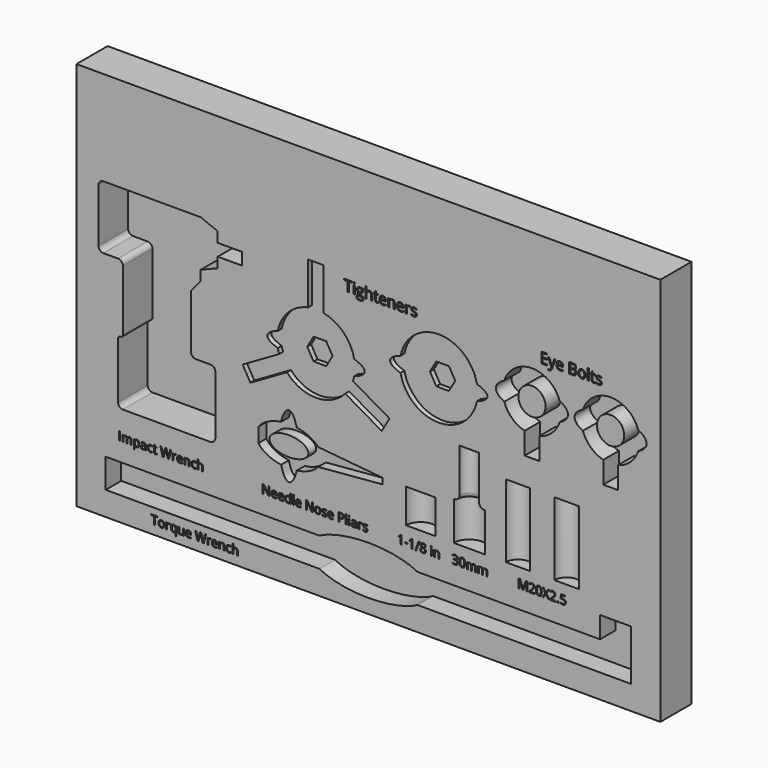
from build123d import *

# Parameters (mm, degrees)
F0_W            = 762
F0_H            = 355.6
F1_DEPTH        = 50.8
F2_R            = 17.78
F3_DEPTH        = 25.4
F0_H_2          = 152.4
F5_DEPTH        = 50.8
F7_DEPTH        = 48.26
F8_DEPTH        = 6.35
F9_DEPTH        = 12.7
F11_DEPTH       = 12.7
F12_DEPTH       = 6.35
F13_DEPTH       = 12.7
F14_TEXT_SIZE   = 15.875
F14_TEXT_SIZE_2 = 19.4027777778
F15_DEPTH       = 3.81
F20_DEPTH       = 12.7
F2_W            = 12.7
F2_H            = 63.5
F22_R           = 6.35


# Not quite as in the source:
# - Text() gives the source's letters only with a copy of the font that has no kerning and outlines rounded to 1/6400 em; it was checked with that copy


with BuildPart() as f1:
    # F0 (on Front) → F1 (new body)
    with BuildSketch(Plane.XZ):
        Rectangle(F0_W, F0_H)
    extrude(amount=F1_DEPTH)

    # F2 (on face) → F3 (cut)
    with BuildSketch(Plane.XZ.offset(50.8)):
        with BuildLine():
            Line((302.26, -80.5533003902), (302.26, -108.4933003902))
            Line((302.26, -108.4933003902), (64.0476572037, -108.4933003902))
            add(Edge.make_bspline(
                [(64.0476572037, -108.4933003902), (0, -74.6266337236), (-64.0476572037, -108.4933003902)],
                knots=[3.7850937624, 3.7850937624, 3.7850937624, 5.6396841984, 5.6396841984, 5.6396841984], degree=2, weights=[1, 0.6, 1]))
            Line((-64.0476572037, -108.4933003902), (-342.9, -108.4933003902))
            Line((-342.9, -108.4933003902), (-342.9, -146.5933003902))
            Line((-342.9, -146.5933003902), (-64.0476572037, -146.5933003902))
            add(Edge.make_bspline(
                [(-64.0476572037, -146.5933003902), (0, -180.4599670569), (64.0476572037, -146.5933003902)],
                knots=[0.6435011088, 0.6435011088, 0.6435011088, 2.4980915448, 2.4980915448, 2.4980915448], degree=2, weights=[1, 0.6, 1]))
            Line((64.0476572037, -146.5933003902), (302.26, -146.5933003902))
            Line((302.26, -146.5933003902), (322.58, -146.5933003902))
            Line((322.58, -146.5933003902), (322.58, -80.5533003902))
            Line((322.58, -80.5533003902), (302.26, -80.5533003902))
        make_face()
        with BuildLine():
            Line((325.5514520794, 70.534063589), (325.5514520794, 99.109063589))
            ThreePointArc((325.5514520794, 99.109063589), (341.9633701455, 108.0906957609), (352.1212254393, 123.8017984246))
            add(Edge.make_bspline(
                [(352.1212254393, 123.8017984246), (377.2004087071, 135.9992299616), (352.1212254393, 148.1966614987)],
                knots=[5.5883159153, 5.5883159153, 5.5883159153, 6.9780546991, 6.9780546991, 6.9780546991], degree=2, weights=[1, 0.7681373347, 1]))
            ThreePointArc((352.1212254393, 148.1966614987), (316.0264520794, 174.0992299616), (279.9316787196, 148.1966614987))
            add(Edge.make_bspline(
                [(279.9316787196, 148.1966614987), (254.8524954518, 135.9992299616), (279.9316787196, 123.8017984246)],
                knots=[2.4467232617, 2.4467232617, 2.4467232617, 3.8364620455, 3.8364620455, 3.8364620455], degree=2, weights=[1, 0.7681373347, 1]))
            ThreePointArc((279.9316787196, 123.8017984246), (290.0895340134, 108.0906957609), (306.5014520794, 99.109063589))
            Line((306.5014520794, 99.109063589), (306.5014520794, 70.534063589))
            Line((306.5014520794, 70.534063589), (316.0264520794, 70.534063589))
            Line((316.0264520794, 70.534063589), (325.5514520794, 70.534063589))
        make_face()
        with BuildLine():
            ThreePointArc((316.0264520794, 118.2192299616), (303.4540935099, 148.5715885311), (333.8064520794, 135.9992299616))
            ThreePointArc((333.8064520794, 135.9992299616), (328.5988106489, 123.4268713921), (316.0264520794, 118.2192299616))
        make_face(mode=Mode.SUBTRACT)
        with BuildLine():
            Line((222.9323361307, 70.534063589), (222.9323361307, 99.109063589))
            ThreePointArc((222.9323361307, 99.109063589), (239.3442541968, 108.0906957609), (249.5021094906, 123.8017984246))
            add(Edge.make_bspline(
                [(249.5021094906, 123.8017984246), (274.5812927584, 135.9992299616), (249.5021094906, 148.1966614987)],
                knots=[2.4467232617, 2.4467232617, 2.4467232617, 3.8364620455, 3.8364620455, 3.8364620455], degree=2, weights=[1, 0.7681373347, 1]))
            ThreePointArc((249.5021094906, 148.1966614987), (213.4073361307, 174.0992299616), (177.3125627709, 148.1966614987))
            add(Edge.make_bspline(
                [(177.3125627709, 148.1966614987), (152.2333795031, 135.9992299616), (177.3125627709, 123.8017984246)],
                knots=[5.5883159153, 5.5883159153, 5.5883159153, 6.9780546991, 6.9780546991, 6.9780546991], degree=2, weights=[1, 0.7681373347, 1]))
            ThreePointArc((177.3125627709, 123.8017984246), (187.4704180647, 108.0906957609), (203.8823361307, 99.109063589))
            Line((203.8823361307, 99.109063589), (203.8823361307, 70.534063589))
            Line((203.8823361307, 70.534063589), (213.4073361307, 70.534063589))
            Line((213.4073361307, 70.534063589), (222.9323361307, 70.534063589))
        make_face()
        with Locations((213.4073361307, 135.9992299616)):
            Circle(F2_R, mode=Mode.SUBTRACT)
        Polygon((342.9, -80.5533003902), (322.58, -80.5533003902), (322.58, -146.5933003902), (342.9, -146.5933003902), (342.9, -108.4933003902), align=None)
    extrude(amount=-F3_DEPTH, mode=Mode.SUBTRACT)

    # F0 (on Front) → F5 (join)
    with BuildSketch(Plane.XZ):
        with Locations((0, 254)):
            Rectangle(F0_W, F0_H_2)
    extrude(amount=F5_DEPTH)

    # F6 (on face) → F7 (cut)
    with BuildSketch(Plane.XZ.offset(50.8)):
        with BuildLine():
            Line((-218.8787088156, 206.9589091301), (-345.8787088156, 206.9589091301))
            ThreePointArc((-345.8787088156, 206.9589091301), (-350.3688368761, 205.0990371906), (-352.2287088156, 200.6089091301))
            Line((-352.2287088156, 200.6089091301), (-352.2287088156, 130.7589091301))
            ThreePointArc((-352.2287088156, 130.7589091301), (-350.3688368761, 126.2687810696), (-345.8787088156, 124.4089091301))
            Line((-345.8787088156, 124.4089091301), (-326.8287088156, 124.4089091301))
            ThreePointArc((-326.8287088156, 124.4089091301), (-322.338580755, 122.5490371906), (-320.4787088156, 118.0589091301))
            Line((-320.4787088156, 118.0589091301), (-320.4787088156, 38.6839091301))
            ThreePointArc((-320.4787088156, 38.6839091301), (-321.4086447853, 36.4388450998), (-323.6537088156, 35.5089091301))
            ThreePointArc((-323.6537088156, 35.5089091301), (-325.8987728458, 34.5789731604), (-326.8287088156, 32.3339091301))
            Line((-326.8287088156, 32.3339091301), (-326.8287088156, -40.6910908699))
            ThreePointArc((-326.8287088156, -40.6910908699), (-324.9688368761, -45.1812189304), (-320.4787088156, -47.0410908699))
            Line((-320.4787088156, -47.0410908699), (-206.1787088156, -47.0410908699))
            ThreePointArc((-206.1787088156, -47.0410908699), (-201.688580755, -45.1812189304), (-199.8287088156, -40.6910908699))
            Line((-199.8287088156, -40.6910908699), (-199.8287088156, 35.5089091301))
            ThreePointArc((-199.8287088156, 35.5089091301), (-201.688580755, 39.9990371906), (-206.1787088156, 41.8589091301))
            Line((-206.1787088156, 41.8589091301), (-225.2287088156, 41.8589091301))
            ThreePointArc((-225.2287088156, 41.8589091301), (-229.7188368761, 43.7187810696), (-231.5787088156, 48.2089091301))
            Line((-231.5787088156, 48.2089091301), (-231.5787088156, 118.0589091301))
            Line((-231.5787088156, 118.0589091301), (-218.8787088156, 133.9339091301))
            Line((-218.8787088156, 133.9339091301), (-218.8787088156, 146.6339091301))
            Line((-218.8787088156, 146.6339091301), (-196.6537088156, 155.5239091301))
            Line((-196.6537088156, 155.5239091301), (-196.6537088156, 168.8589091301))
            Line((-196.6537088156, 168.8589091301), (-164.9037088156, 168.8589091301))
            Line((-164.9037088156, 168.8589091301), (-164.9037088156, 184.7339091301))
            Line((-164.9037088156, 184.7339091301), (-196.6537088156, 184.7339091301))
            Line((-196.6537088156, 184.7339091301), (-196.6537088156, 198.0689091301))
            Line((-196.6537088156, 198.0689091301), (-218.8787088156, 206.9589091301))
        make_face()
    extrude(amount=-F7_DEPTH, mode=Mode.SUBTRACT)

    # F6 (on face) → F8 (cut)
    with BuildSketch(Plane.XZ.offset(50.8)):
        with BuildLine():
            add(Edge.make_bspline(
                [(-118.2285690843, 109.0660422975), (-149.2966618743, 99.2286645982), (-118.2285690843, 89.3912868988)],
                knots=[2.4732611299, 2.4732611299, 2.4732611299, 3.8099241773, 3.8099241773, 3.8099241773], degree=2, weights=[1, 0.7848566748, 1]))
            ThreePointArc((-118.2285690843, 89.3912868988), (-117.4795035517, 86.1566580811), (-116.520739255, 82.9778699814))
            Line((-116.520739255, 82.9778699814), (-164.1237066018, 55.4942839694))
            Line((-164.1237066018, 55.4942839694), (-159.0437066018, 46.695465867))
            Line((-159.0437066018, 46.695465867), (-153.9637066018, 37.8966477645))
            Line((-153.9637066018, 37.8966477645), (-106.3012300457, 65.4145914345))
            ThreePointArc((-106.3012300457, 65.4145914345), (-68.2183829259, 48.4289550604), (-30.2512847531, 65.6717664354))
            Line((-30.2512847531, 65.6717664354), (17.3516825938, 38.1881804235))
            Line((17.3516825938, 38.1881804235), (22.4316825938, 46.9869985259))
            Line((22.4316825938, 46.9869985259), (27.5116825938, 55.7858166284))
            Line((27.5116825938, 55.7858166284), (-20.1507939623, 83.3037602983))
            ThreePointArc((-20.1507939623, 83.3037602983), (-19.2569127775, 86.3227352727), (-18.5517713829, 89.3912868988))
            add(Edge.make_bspline(
                [(-18.5517713829, 89.3912868988), (12.5163214072, 99.2286645982), (-18.5517713829, 109.0660422975)],
                knots=[5.6148537835, 5.6148537835, 5.6148537835, 6.9515168309, 6.9515168309, 6.9515168309], degree=2, weights=[1, 0.7848566748, 1]))
            ThreePointArc((-18.5517713829, 109.0660422975), (-32.4135637837, 135.0940209794), (-58.3984866927, 149.0363573777))
            Line((-58.3984866927, 149.0363573777), (-58.3984866927, 204.0035294015))
            Line((-58.3984866927, 204.0035294015), (-68.5584866927, 204.0035294015))
            Line((-68.5584866927, 204.0035294015), (-78.7184866927, 204.0035294015))
            Line((-78.7184866927, 204.0035294015), (-78.7184866927, 148.9676420617))
            ThreePointArc((-78.7184866927, 148.9676420617), (-104.4878546985, 134.9721559815), (-118.2285690843, 109.0660422975))
        make_face()
        Polygon((-68.3901702336, 113.5161748096), (-60.1242022144, 113.5062921219), (-51.8923980827, 99.2089400686), (-60.1583661018, 84.9313125448), (-76.6561382527, 84.9510370744), (-84.8879423845, 99.2483891277), (-76.6219743653, 113.5260166515), align=None, mode=Mode.SUBTRACT)
    extrude(amount=-F8_DEPTH, mode=Mode.SUBTRACT)

    # F6 (on face) → F9 (cut)
    with BuildSketch(Plane.XZ.offset(50.8)):
        Polygon((-51.8923980827, 99.2089400686), (-60.1242022144, 113.5062921219), (-68.3901702336, 113.5161748096), (-76.6219743653, 113.5260166515), (-84.8879423845, 99.2483891277), (-76.6561382527, 84.9510370744), (-60.1583661018, 84.9313125448), align=None)
    extrude(amount=-F9_DEPTH, mode=Mode.SUBTRACT)

    # F10 (on face) → F11 (cut)
    with BuildSketch(Plane.XZ.offset(50.8)):
        with BuildLine():
            Line((-65.5816475336, -30.0850472887), (18.5110562313, -22.833929086))
            Line((18.5110562313, -22.833929086), (18.5110562313, -19.023929086))
            Line((18.5110562313, -19.023929086), (18.5110562313, -15.213929086))
            Line((18.5110562313, -15.213929086), (-65.5816475336, -7.2250472887))
            add(Edge.make_bspline(
                [(-65.5816475336, -7.2250472887), (-74.4495671038, 3.2276411288), (-93.5893307929, 6.0144929834)],
                knots=[0.466765339, 0.466765339, 0.466765339, 1.3303918197, 1.3303918197, 1.3303918197], degree=2, weights=[1, 0.9082083689, 1]))
            add(Edge.make_bspline(
                [(-93.5893307929, 6.0144929834), (-103.7712937651, 50.4028113586), (-113.9532567372, 6.0144929834)],
                knots=[5.3530022456, 5.3530022456, 5.3530022456, 7.2133683688, 7.2133683688, 7.2133683688], degree=2, weights=[1, 0.5976872265, 1]))
            add(Edge.make_bspline(
                [(-113.9532567372, 6.0144929834), (-135.1024926256, 2.9350512402), (-143.3497070609, -9.035078524)],
                knots=[1.8112008339, 1.8112008339, 1.8112008339, 2.7531593172, 2.7531593172, 2.7531593172], degree=2, weights=[1, 0.8911243757, 1]))
            Line((-143.3497070609, -9.035078524), (-143.4793644948, -28.084637284))
            add(Edge.make_bspline(
                [(-143.4793644948, -28.084637284), (-135.3143735367, -40.2142948249), (-113.9532567372, -43.3245875607)],
                knots=[3.521940738, 3.521940738, 3.521940738, 4.4719844733, 4.4719844733, 4.4719844733], degree=2, weights=[1, 0.8892827205, 1]))
            add(Edge.make_bspline(
                [(-113.9532567372, -43.3245875607), (-103.7712937651, -87.7129059359), (-93.5893307929, -43.3245875607)],
                knots=[2.211409592, 2.211409592, 2.211409592, 4.0717757152, 4.0717757152, 4.0717757152], degree=2, weights=[1, 0.5976872265, 1]))
            add(Edge.make_bspline(
                [(-93.5893307929, -43.3245875607), (-74.4495671038, -40.5377357061), (-65.5816475336, -30.0850472887)],
                knots=[4.9527934875, 4.9527934875, 4.9527934875, 5.8164199681, 5.8164199681, 5.8164199681], degree=2, weights=[1, 0.9082083689, 1]))
        make_face()
        with BuildLine():
            add(Edge.make_bspline(
                [(-78.3712937651, -18.6550472887), (-78.3712937651, 3.3419979675), (-116.4712937651, -7.6565246606), (-154.5712937651, -18.6550472887), (-116.4712937651, -29.6535699167), (-78.3712937651, -40.6520925448), (-78.3712937651, -18.6550472887)],
                knots=[0, 0, 0, 2.0943951024, 2.0943951024, 4.1887902048, 4.1887902048, 6.2831853072, 6.2831853072, 6.2831853072], degree=2, weights=[1, 0.5, 1, 0.5, 1, 0.5, 1]))
        make_face(mode=Mode.SUBTRACT)
    extrude(amount=-F11_DEPTH, mode=Mode.SUBTRACT)

    # F4 (on face) → F12 (cut)
    with BuildSketch(Plane.XZ.offset(50.8)):
        with BuildLine():
            add(Edge.make_bspline(
                [(41.902179652, 132.5469361757), (10.834086862, 122.7095584763), (41.902179652, 112.872180777)],
                knots=[2.4732611299, 2.4732611299, 2.4732611299, 3.8099241773, 3.8099241773, 3.8099241773], degree=2, weights=[1, 0.7848566748, 1]))
            ThreePointArc((41.902179652, 112.872180777), (91.7405785027, 71.9095584763), (141.5789773534, 112.872180777))
            add(Edge.make_bspline(
                [(141.5789773534, 112.872180777), (172.6470701434, 122.7095584763), (141.5789773534, 132.5469361757)],
                knots=[5.6148537835, 5.6148537835, 5.6148537835, 6.9515168309, 6.9515168309, 6.9515168309], degree=2, weights=[1, 0.7848566748, 1]))
            ThreePointArc((141.5789773534, 132.5469361757), (91.7405785027, 173.5095584763), (41.902179652, 132.5469361757))
        make_face()
        Polygon((83.508774371, 137.0069105296), (100.0065465219, 136.987186), (108.2383506536, 122.6898339468), (99.9723826345, 108.412206423), (83.4746104836, 108.4319309526), (75.2428063518, 122.7292830059), align=None, mode=Mode.SUBTRACT)
    extrude(amount=-F12_DEPTH, mode=Mode.SUBTRACT)

    # F13 (cut): a face of the model
    f13_faces = [f1.faces().sort_by_distance(p)[0] for p in [
        (91.7405785027, -50.8, 122.7095584763),
    ]]
    extrude(f13_faces, amount=-F13_DEPTH, mode=Mode.SUBTRACT)

    # F14 (on face) → F15 (cut)
    with BuildSketch(Plane.XZ.offset(50.8)):
        with Locations((-283.68992402, -166.411831975)):
            Text('Torque Wrench', F14_TEXT_SIZE, font='Open Sans', text_align=(TextAlign.LEFT, TextAlign.BOTTOM))
        with Locations((-139.4941210937, -84.4243631911)):
            Text('Needle Nose Pliars', F14_TEXT_SIZE, font='Open Sans', text_align=(TextAlign.LEFT, TextAlign.BOTTOM))
        with Locations((108.8420884107, -84.4243631911)):
            Text('30mm', F14_TEXT_SIZE, font='Open Sans', text_align=(TextAlign.LEFT, TextAlign.BOTTOM))
        with Locations((37.7088141466, -84.4243631911)):
            Text('1-1/8 in', F14_TEXT_SIZE, font='Open Sans', text_align=(TextAlign.LEFT, TextAlign.BOTTOM))
        with Locations((223.6330280026, 183.4626990706)):
            Text('Eye Bolts', F14_TEXT_SIZE_2, font='Open Sans', text_align=(TextAlign.LEFT, TextAlign.BOTTOM))
        with Locations((194.5427989624, -84.4243631911)):
            Text('M20X2.5', F14_TEXT_SIZE, font='Open Sans', text_align=(TextAlign.LEFT, TextAlign.BOTTOM))
        with Locations((-31.7948177179, 183.4626990706)):
            Text('Tighteners', F14_TEXT_SIZE_2, font='Open Sans', text_align=(TextAlign.LEFT, TextAlign.BOTTOM))
        with Locations((-326.8163032341, -84.4243631911)):
            Text('Impact Wrench', F14_TEXT_SIZE, font='Open Sans', text_align=(TextAlign.LEFT, TextAlign.BOTTOM))
    extrude(amount=-F15_DEPTH, mode=Mode.SUBTRACT)

    # F2 (on face) → F16 (revolve, cut)
    with BuildSketch(Plane.XZ.offset(50.8)):
        Polygon((68.1681612015, -59.8321110725), (68.1681612015, -15.3821110725), (49.1181612015, -15.3821110725), (49.1181612015, -29.2827303602), (49.1181612015, -55.1231727004), (49.1181612015, -59.8321110725), align=None)
    revolve(axis=Axis((68.1681612015, -50.8, -37.6071110725), (0, 0, -1)), mode=Mode.SUBTRACT)

    # F2 (on face) → F17 (revolve, cut)
    with BuildSketch(Plane.XZ.offset(50.8)):
        Polygon((195.1681612015, -59.8321110725), (195.1681612015, 35.4178889275), (179.2931612015, 35.4178889275), (179.2931612015, 23.4812485351), (179.2931612015, -1.9259535582), (179.2931612015, -24.7715493716), (179.2931612015, -49.5437514649), (179.2931612015, -59.8321110725), align=None)
    revolve(axis=Axis((195.1681612015, -50.8, -12.2071110725), (0, 0, -1)), mode=Mode.SUBTRACT)

    # F2 (on face) → F18 (revolve, cut)
    with BuildSketch(Plane.XZ.offset(50.8)):
        Polygon((258.6681612015, -59.8321110725), (258.6681612015, 35.4178889275), (242.7931612015, 35.4178889275), (242.7931612015, 3.7906940208), (242.7931612015, -1.9259535582), (242.7931612015, -24.7715493716), (242.7931612015, -30.4881969506), (242.7931612015, -59.8321110725), align=None)
    revolve(axis=Axis((258.6681612015, -50.8, -12.2071110725), (0, 0, -1)), mode=Mode.SUBTRACT)

    # F19 (on face) → F20 (cut)
    with BuildSketch(Plane(origin=(0, 0, 0), x_dir=(-1, 0, 0), z_dir=(0, 1, 0))):
        with BuildLine():
            ThreePointArc((279.4, -155.575), (295.275, -139.7), (279.4, -123.825))
            Line((279.4, -123.825), (0, -123.825))
            Line((0, -123.825), (-279.4, -123.825))
            ThreePointArc((-279.4, -123.825), (-295.275, -139.7), (-279.4, -155.575))
            Line((-279.4, -155.575), (279.4, -155.575))
        make_face()
    extrude(amount=-F20_DEPTH, mode=Mode.SUBTRACT)

    # F2 (on face) → F21 (revolve, cut)
    with BuildSketch(Plane.XZ.offset(50.8)):
        Polygon((131.6681612015, -59.8321110725), (131.6681612015, -9.0321110725), (118.9681612015, -9.0321110725), (111.3481612015, -9.0321110725), (111.3481612015, -29.1846399694), (111.3481612015, -47.0428629604), (111.3481612015, -59.8321110725), align=None)
        with Locations((125.3181612015, 22.7178889275)):
            Rectangle(F2_W, F2_H)
    revolve(axis=Axis((131.6681612015, -50.8, -2.6821110725), (0, 0, -1)), mode=Mode.SUBTRACT)

    # F22
    f22_edges = [f1.edges().sort_by_distance(p)[0] for p in [
        (131.668161, -38.1, -9.032111),
    ]]
    fillet(f22_edges, radius=F22_R)


solid = f1.part
